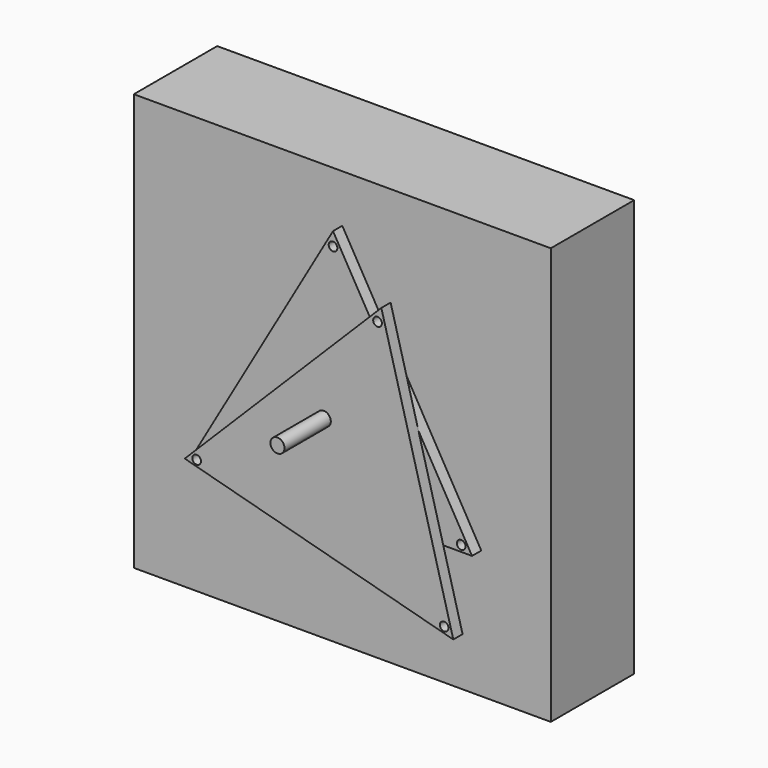
from build123d import *

# Parameters (mm, degrees)
F0_R     = 9.525
F2_DEPTH = 25.4
F1_R     = 9.525
F3_DEPTH = 25.4
F5_START = -25.4
F4_W     = 914.4
F4_H     = 914.4
F4_R     = 15.448541342
F5_DEPTH = 228.6
F6_DEPTH = 152.4


with BuildPart() as f2:
    # F0 (on Front) → F2 (new body)
    with BuildSketch(Plane.XZ):
        Polygon((-304.8, -175.976362049), (304.8, -175.976362049), (0, 351.952724098), align=None)
        with Locations((-280.8323993128, -162.1386613404)):
            Circle(F0_R, mode=Mode.SUBTRACT)
        with Locations((281.140565359, -162.3165810902)):
            Circle(F0_R, mode=Mode.SUBTRACT)
        with Locations((0, 322.2702741623)):
            Circle(F0_R, mode=Mode.SUBTRACT)
    extrude(amount=-F2_DEPTH)


with BuildPart() as f3:
    # F1 (on face) → F3 (new body)
    with BuildSketch(Plane.XZ):
        Polygon((-304.8, -175.976362049), (284.0283837058, -333.7524519435), (126.2522938113, 255.0759317623), align=None)
        with Locations((-278.7650227547, -169.6263700724)):
            Circle(F1_R, mode=Mode.SUBTRACT)
        with Locations((264.0131284784, -315.2475334434)):
            Circle(F1_R, mode=Mode.SUBTRACT)
        with Locations((117.8725027263, 225.5919577909)):
            Circle(F1_R, mode=Mode.SUBTRACT)
    extrude(amount=F3_DEPTH)


with BuildPart() as f5:
    # F4 (on Front) → F5 (new body)
    with BuildSketch(Plane.XZ.offset(F5_START)):
        Rectangle(F4_W, F4_H)
        Circle(F4_R, mode=Mode.SUBTRACT)
    extrude(amount=-F5_DEPTH)


with BuildPart() as f6:
    # F4 (on Front) → F6 (new body)
    with BuildSketch(Plane.XZ):
        Circle(F4_R)
    extrude(amount=F6_DEPTH)


solid = Compound([f2.part, f3.part, f5.part, f6.part])
